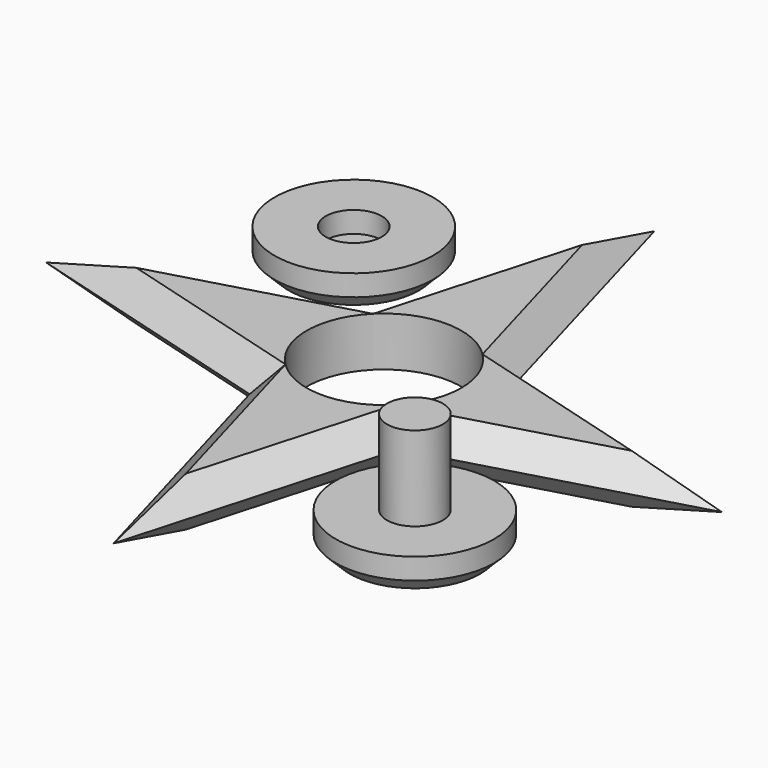
from build123d import *

# Parameters (mm, degrees)
F0_R          = 11
F1_DEPTH      = 7
F2_T4_DEPTH   = 56.8703573637
F2_T9_DEPTH   = 56.8703573637
F2_T14_DEPTH  = 56.8703573637
F2_T19_DEPTH  = 56.8703573637
F2_T24_DEPTH  = 56.8703573637
F2_T29_DEPTH  = 56.8703573637
F2_T34_DEPTH  = 56.8703573637
F2_T39_DEPTH  = 56.8703573637
F2_T44_DEPTH  = 56.8703573637
F2_T49_DEPTH  = 56.8703573637
F2_T54_DEPTH  = 56.8703573637
F2_T59_DEPTH  = 56.8703573637
F2_T64_DEPTH  = 56.8703573637
F2_T69_DEPTH  = 56.8703573637
F2_T74_DEPTH  = 56.8703573637
F2_T79_DEPTH  = 56.8703573637
F2_T85_DEPTH  = 56.8703573637
F2_T89_DEPTH  = 56.8703573637
F2_T96_DEPTH  = 56.8703573637
F2_T100_DEPTH = 56.8703573637
F2_T107_DEPTH = 56.8703573637
F2_T111_DEPTH = 56.8703573637
F2_T118_DEPTH = 56.8703573637
F2_T122_DEPTH = 56.8703573637
F2_T129_DEPTH = 56.8703573637
F2_T133_DEPTH = 56.8703573637
F2_T140_DEPTH = 56.8703573637
F2_T144_DEPTH = 56.8703573637
F2_T151_DEPTH = 56.8703573637
F2_T155_DEPTH = 56.8703573637
F2_T162_DEPTH = 56.8703573637
F2_T166_DEPTH = 56.8703573637
F3_R          = 11.25
F4_DEPTH      = 5
F5_R          = 3.98
F6_DEPTH      = 12
F7_SIZE       = 2
F8_R          = 11.25
F9_DEPTH      = 5
F10_R         = 3.98
F11_DEPTH     = 3
F12_SIZE      = 2


# Not quite as in the source:
# - a fillet or chamfer that OpenCascade refuses, or shapes differently, is made with other operations: its cross-section is extruded or revolved along the edge and cut away or added


with BuildPart() as f1:
    # F0 (on Top) → F1 (new body)
    with BuildSketch(Plane.XY):
        Polygon((-10.6066017178, 10.6066017178), (-48, 0), (-10.6066017178, -10.6066017178), (0, -48), (10.6066017178, -10.6066017178), (48, 0), (10.6066017178, 10.6066017178), (0, 48), align=None)
        Circle(F0_R, mode=Mode.SUBTRACT)
    extrude(amount=F1_DEPTH)

    # F2: chamfer of 3.5 on 16 edges, made by hand


with BuildPart() as f2_tool2:
    # F2_s3 → F2_t4 (new body)
    with BuildSketch(Plane(origin=(15.0574910401, 53.0849347014, 0), x_dir=(0, 0, 1), z_dir=(-0.2728837196, -0.9620470236, 0))):
        Polygon((3.5, 13.0984185422), (7, 9.5984185422), (7, 13.0984185422), align=None)
    extrude(amount=F2_T4_DEPTH)

    split(bisect_by=Plane(origin=(-3.574345173, 12.601294572, 0), x_dir=(0, 0, 1), z_dir=(-0.2728837196, 0.9620470236, 0)), keep=Keep.TOP)


with BuildPart() as f1_1:
    add(f1.part)

    # F2_t1: cut F2_tool2
    add(f2_tool2.part, mode=Mode.SUBTRACT)


with BuildPart() as f2_tool7:
    # F2_s8 → F2_t9 (new body)
    with BuildSketch(Plane(origin=(0.4615036139, -1.6270233297, 0), x_dir=(0, 0, 1), z_dir=(-0.2728837196, 0.9620470236, 0))):
        Polygon((3.5, 13.0984185422), (7, 9.5984185422), (7, 13.0984185422), align=None)
    extrude(amount=F2_T9_DEPTH)

    split(bisect_by=Plane(origin=(3.574345173, 12.601294572, 0), x_dir=(0, 0, 1), z_dir=(0.2728837196, 0.9620470236, 0)), keep=Keep.TOP)


with BuildPart() as f1_2:
    add(f1_1.part)

    # F2_t6: cut F2_tool7
    add(f2_tool7.part, mode=Mode.SUBTRACT)


with BuildPart() as f2_tool12:
    # F2_s13 → F2_t14 (new body)
    with BuildSketch(Plane(origin=(53.0849347014, -15.0574910401, 0), x_dir=(0, 0, 1), z_dir=(-0.9620470236, 0.2728837196, 0))):
        Polygon((3.5, 13.0984185422), (7, 9.5984185422), (7, 13.0984185422), align=None)
    extrude(amount=F2_T14_DEPTH)

    split(bisect_by=Plane(origin=(12.601294572, 3.574345173, 0), x_dir=(0, 0, 1), z_dir=(0.9620470236, 0.2728837196, 0)), keep=Keep.TOP)


with BuildPart() as f1_3:
    add(f1_2.part)

    # F2_t11: cut F2_tool12
    add(f2_tool12.part, mode=Mode.SUBTRACT)


with BuildPart() as f2_tool17:
    # F2_s18 → F2_t19 (new body)
    with BuildSketch(Plane(origin=(-1.6270233297, -0.4615036139, 0), x_dir=(0, 0, 1), z_dir=(0.9620470236, 0.2728837196, 0))):
        Polygon((3.5, 13.0984185422), (7, 9.5984185422), (7, 13.0984185422), align=None)
    extrude(amount=F2_T19_DEPTH)

    split(bisect_by=Plane(origin=(12.601294572, -3.574345173, 0), x_dir=(0, 0, 1), z_dir=(0.9620470236, -0.2728837196, 0)), keep=Keep.TOP)


with BuildPart() as f1_4:
    add(f1_3.part)

    # F2_t16: cut F2_tool17
    add(f2_tool17.part, mode=Mode.SUBTRACT)


with BuildPart() as f2_tool22:
    # F2_s23 → F2_t24 (new body)
    with BuildSketch(Plane(origin=(-15.0574910401, -53.0849347014, 0), x_dir=(0, 0, 1), z_dir=(0.2728837196, 0.9620470236, 0))):
        Polygon((3.5, 13.0984185422), (7, 9.5984185422), (7, 13.0984185422), align=None)
    extrude(amount=F2_T24_DEPTH)

    split(bisect_by=Plane(origin=(3.574345173, -12.601294572, 0), x_dir=(0, 0, 1), z_dir=(0.2728837196, -0.9620470236, 0)), keep=Keep.TOP)


with BuildPart() as f1_5:
    add(f1_4.part)

    # F2_t21: cut F2_tool22
    add(f2_tool22.part, mode=Mode.SUBTRACT)


with BuildPart() as f2_tool27:
    # F2_s28 → F2_t29 (new body)
    with BuildSketch(Plane(origin=(-0.4615036139, 1.6270233297, 0), x_dir=(0, 0, 1), z_dir=(0.2728837196, -0.9620470236, 0))):
        Polygon((3.5, 13.0984185422), (7, 9.5984185422), (7, 13.0984185422), align=None)
    extrude(amount=F2_T29_DEPTH)

    split(bisect_by=Plane(origin=(-3.574345173, -12.601294572, 0), x_dir=(0, 0, 1), z_dir=(-0.2728837196, -0.9620470236, 0)), keep=Keep.TOP)


with BuildPart() as f1_6:
    add(f1_5.part)

    # F2_t26: cut F2_tool27
    add(f2_tool27.part, mode=Mode.SUBTRACT)


with BuildPart() as f2_tool32:
    # F2_s33 → F2_t34 (new body)
    with BuildSketch(Plane(origin=(-53.0849347014, 15.0574910401, 0), x_dir=(0, 0, 1), z_dir=(0.9620470236, -0.2728837196, 0))):
        Polygon((3.5, 13.0984185422), (7, 9.5984185422), (7, 13.0984185422), align=None)
    extrude(amount=F2_T34_DEPTH)

    split(bisect_by=Plane(origin=(-12.601294572, -3.574345173, 0), x_dir=(0, 0, 1), z_dir=(-0.9620470236, -0.2728837196, 0)), keep=Keep.TOP)


with BuildPart() as f1_7:
    add(f1_6.part)

    # F2_t31: cut F2_tool32
    add(f2_tool32.part, mode=Mode.SUBTRACT)


with BuildPart() as f2_tool37:
    # F2_s38 → F2_t39 (new body)
    with BuildSketch(Plane(origin=(1.6270233297, 0.4615036139, 0), x_dir=(0, 0, 1), z_dir=(-0.9620470236, -0.2728837196, 0))):
        Polygon((3.5, 13.0984185422), (7, 9.5984185422), (7, 13.0984185422), align=None)
    extrude(amount=F2_T39_DEPTH)

    split(bisect_by=Plane(origin=(-12.601294572, 3.574345173, 0), x_dir=(0, 0, 1), z_dir=(-0.9620470236, 0.2728837196, 0)), keep=Keep.TOP)


with BuildPart() as f1_8:
    add(f1_7.part)

    # F2_t36: cut F2_tool37
    add(f2_tool37.part, mode=Mode.SUBTRACT)


with BuildPart() as f2_tool42:
    # F2_s43 → F2_t44 (new body)
    with BuildSketch(Plane(origin=(-53.0849347014, 15.0574910401, 0), x_dir=(0, 0, 1), z_dir=(0.9620470236, -0.2728837196, 0))):
        Polygon((3.5, 13.0984185422), (0, 9.5984185422), (0, 13.0984185422), align=None)
    extrude(amount=F2_T44_DEPTH)

    split(bisect_by=Plane(origin=(-12.601294572, -3.574345173, 0), x_dir=(0, 0, 1), z_dir=(-0.9620470236, -0.2728837196, 0)), keep=Keep.TOP)


with BuildPart() as f1_9:
    add(f1_8.part)

    # F2_t41: cut F2_tool42
    add(f2_tool42.part, mode=Mode.SUBTRACT)


with BuildPart() as f2_tool47:
    # F2_s48 → F2_t49 (new body)
    with BuildSketch(Plane(origin=(1.6270233297, 0.4615036139, 0), x_dir=(0, 0, 1), z_dir=(-0.9620470236, -0.2728837196, 0))):
        Polygon((3.5, 13.0984185422), (0, 9.5984185422), (0, 13.0984185422), align=None)
    extrude(amount=F2_T49_DEPTH)

    split(bisect_by=Plane(origin=(-12.601294572, 3.574345173, 0), x_dir=(0, 0, 1), z_dir=(-0.9620470236, 0.2728837196, 0)), keep=Keep.TOP)


with BuildPart() as f1_10:
    add(f1_9.part)

    # F2_t46: cut F2_tool47
    add(f2_tool47.part, mode=Mode.SUBTRACT)


with BuildPart() as f2_tool52:
    # F2_s53 → F2_t54 (new body)
    with BuildSketch(Plane(origin=(15.0574910401, 53.0849347014, 0), x_dir=(0, 0, 1), z_dir=(-0.2728837196, -0.9620470236, 0))):
        Polygon((3.5, 13.0984185422), (0, 9.5984185422), (0, 13.0984185422), align=None)
    extrude(amount=F2_T54_DEPTH)

    split(bisect_by=Plane(origin=(-3.574345173, 12.601294572, 0), x_dir=(0, 0, 1), z_dir=(-0.2728837196, 0.9620470236, 0)), keep=Keep.TOP)


with BuildPart() as f1_11:
    add(f1_10.part)

    # F2_t51: cut F2_tool52
    add(f2_tool52.part, mode=Mode.SUBTRACT)


with BuildPart() as f2_tool57:
    # F2_s58 → F2_t59 (new body)
    with BuildSketch(Plane(origin=(-0.4615036139, 1.6270233297, 0), x_dir=(0, 0, 1), z_dir=(0.2728837196, -0.9620470236, 0))):
        Polygon((3.5, 13.0984185422), (0, 9.5984185422), (0, 13.0984185422), align=None)
    extrude(amount=F2_T59_DEPTH)

    split(bisect_by=Plane(origin=(-3.574345173, -12.601294572, 0), x_dir=(0, 0, 1), z_dir=(-0.2728837196, -0.9620470236, 0)), keep=Keep.TOP)


with BuildPart() as f1_12:
    add(f1_11.part)

    # F2_t56: cut F2_tool57
    add(f2_tool57.part, mode=Mode.SUBTRACT)


with BuildPart() as f2_tool62:
    # F2_s63 → F2_t64 (new body)
    with BuildSketch(Plane(origin=(-15.0574910401, -53.0849347014, 0), x_dir=(0, 0, 1), z_dir=(0.2728837196, 0.9620470236, 0))):
        Polygon((3.5, 13.0984185422), (0, 9.5984185422), (0, 13.0984185422), align=None)
    extrude(amount=F2_T64_DEPTH)

    split(bisect_by=Plane(origin=(3.574345173, -12.601294572, 0), x_dir=(0, 0, 1), z_dir=(0.2728837196, -0.9620470236, 0)), keep=Keep.TOP)


with BuildPart() as f1_13:
    add(f1_12.part)

    # F2_t61: cut F2_tool62
    add(f2_tool62.part, mode=Mode.SUBTRACT)


with BuildPart() as f2_tool67:
    # F2_s68 → F2_t69 (new body)
    with BuildSketch(Plane(origin=(-1.6270233297, -0.4615036139, 0), x_dir=(0, 0, 1), z_dir=(0.9620470236, 0.2728837196, 0))):
        Polygon((3.5, 13.0984185422), (0, 9.5984185422), (0, 13.0984185422), align=None)
    extrude(amount=F2_T69_DEPTH)

    split(bisect_by=Plane(origin=(12.601294572, -3.574345173, 0), x_dir=(0, 0, 1), z_dir=(0.9620470236, -0.2728837196, 0)), keep=Keep.TOP)


with BuildPart() as f1_14:
    add(f1_13.part)

    # F2_t66: cut F2_tool67
    add(f2_tool67.part, mode=Mode.SUBTRACT)


with BuildPart() as f2_tool72:
    # F2_s73 → F2_t74 (new body)
    with BuildSketch(Plane(origin=(53.0849347014, -15.0574910401, 0), x_dir=(0, 0, 1), z_dir=(-0.9620470236, 0.2728837196, 0))):
        Polygon((3.5, 13.0984185422), (0, 9.5984185422), (0, 13.0984185422), align=None)
    extrude(amount=F2_T74_DEPTH)

    split(bisect_by=Plane(origin=(12.601294572, 3.574345173, 0), x_dir=(0, 0, 1), z_dir=(0.9620470236, 0.2728837196, 0)), keep=Keep.TOP)


with BuildPart() as f1_15:
    add(f1_14.part)

    # F2_t71: cut F2_tool72
    add(f2_tool72.part, mode=Mode.SUBTRACT)


with BuildPart() as f2_tool77:
    # F2_s78 → F2_t79 (new body)
    with BuildSketch(Plane(origin=(0.4615036139, -1.6270233297, 0), x_dir=(0, 0, 1), z_dir=(-0.2728837196, 0.9620470236, 0))):
        Polygon((3.5, 13.0984185422), (0, 9.5984185422), (0, 13.0984185422), align=None)
    extrude(amount=F2_T79_DEPTH)

    split(bisect_by=Plane(origin=(3.574345173, 12.601294572, 0), x_dir=(0, 0, 1), z_dir=(0.2728837196, 0.9620470236, 0)), keep=Keep.TOP)


with BuildPart() as f1_16:
    add(f1_15.part)

    # F2_t76: cut F2_tool77
    add(f2_tool77.part, mode=Mode.SUBTRACT)


with BuildPart() as f2_tool83:
    # F2_s84 → F2_t85 (new body)
    with BuildSketch(Plane(origin=(1.6270233297, 0.4615036139, 0), x_dir=(0, 0, 1), z_dir=(-0.9620470236, -0.2728837196, 0))):
        Polygon((3.5, 13.0984185422), (7, 9.5984185422), (7, 13.0984185422), align=None)
    extrude(amount=F2_T85_DEPTH)

    split(bisect_by=Plane(origin=(-12.601294572, 3.574345173, 0), x_dir=(0, 0, 1), z_dir=(0.9620470236, -0.2728837196, 0)), keep=Keep.TOP)


with BuildPart() as f2_tool87:
    # F2_s88 → F2_t89 (new body)
    with BuildSketch(Plane(origin=(15.0574910401, 53.0849347014, 0), x_dir=(0, 0, 1), z_dir=(-0.2728837196, -0.9620470236, 0))):
        Polygon((3.5, 13.0984185422), (7, 9.5984185422), (7, 13.0984185422), align=None)
    extrude(amount=F2_T89_DEPTH)

    split(bisect_by=Plane(origin=(-3.574345173, 12.601294572, 0), x_dir=(0, 0, 1), z_dir=(0.2728837196, -0.9620470236, 0)), keep=Keep.TOP)


with BuildPart() as f2_tool83_1:
    add(f2_tool83.part)

    # F2_t91: intersect F2_tool87
    add(f2_tool87.part, mode=Mode.INTERSECT)


with BuildPart() as f1_17:
    add(f1_16.part)

    # F2_t81: cut F2_tool83
    add(f2_tool83_1.part, mode=Mode.SUBTRACT)


with BuildPart() as f2_tool94:
    # F2_s95 → F2_t96 (new body)
    with BuildSketch(Plane(origin=(53.0849347014, -15.0574910401, 0), x_dir=(0, 0, 1), z_dir=(-0.9620470236, 0.2728837196, 0))):
        Polygon((3.5, 13.0984185422), (7, 9.5984185422), (7, 13.0984185422), align=None)
    extrude(amount=F2_T96_DEPTH)

    split(bisect_by=Plane(origin=(12.601294572, 3.574345173, 0), x_dir=(0, 0, 1), z_dir=(-0.9620470236, -0.2728837196, 0)), keep=Keep.TOP)


with BuildPart() as f2_tool98:
    # F2_s99 → F2_t100 (new body)
    with BuildSketch(Plane(origin=(0.4615036139, -1.6270233297, 0), x_dir=(0, 0, 1), z_dir=(-0.2728837196, 0.9620470236, 0))):
        Polygon((3.5, 13.0984185422), (7, 9.5984185422), (7, 13.0984185422), align=None)
    extrude(amount=F2_T100_DEPTH)

    split(bisect_by=Plane(origin=(3.574345173, 12.601294572, 0), x_dir=(0, 0, 1), z_dir=(-0.2728837196, -0.9620470236, 0)), keep=Keep.TOP)


with BuildPart() as f2_tool94_1:
    add(f2_tool94.part)

    # F2_t102: intersect F2_tool98
    add(f2_tool98.part, mode=Mode.INTERSECT)


with BuildPart() as f1_18:
    add(f1_17.part)

    # F2_t92: cut F2_tool94
    add(f2_tool94_1.part, mode=Mode.SUBTRACT)


with BuildPart() as f2_tool105:
    # F2_s106 → F2_t107 (new body)
    with BuildSketch(Plane(origin=(-15.0574910401, -53.0849347014, 0), x_dir=(0, 0, 1), z_dir=(0.2728837196, 0.9620470236, 0))):
        Polygon((3.5, 13.0984185422), (7, 9.5984185422), (7, 13.0984185422), align=None)
    extrude(amount=F2_T107_DEPTH)

    split(bisect_by=Plane(origin=(3.574345173, -12.601294572, 0), x_dir=(0, 0, 1), z_dir=(-0.2728837196, 0.9620470236, 0)), keep=Keep.TOP)


with BuildPart() as f2_tool109:
    # F2_s110 → F2_t111 (new body)
    with BuildSketch(Plane(origin=(-1.6270233297, -0.4615036139, 0), x_dir=(0, 0, 1), z_dir=(0.9620470236, 0.2728837196, 0))):
        Polygon((3.5, 13.0984185422), (7, 9.5984185422), (7, 13.0984185422), align=None)
    extrude(amount=F2_T111_DEPTH)

    split(bisect_by=Plane(origin=(12.601294572, -3.574345173, 0), x_dir=(0, 0, 1), z_dir=(-0.9620470236, 0.2728837196, 0)), keep=Keep.TOP)


with BuildPart() as f2_tool105_1:
    add(f2_tool105.part)

    # F2_t113: intersect F2_tool109
    add(f2_tool109.part, mode=Mode.INTERSECT)


with BuildPart() as f1_19:
    add(f1_18.part)

    # F2_t103: cut F2_tool105
    add(f2_tool105_1.part, mode=Mode.SUBTRACT)


with BuildPart() as f2_tool116:
    # F2_s117 → F2_t118 (new body)
    with BuildSketch(Plane(origin=(-53.0849347014, 15.0574910401, 0), x_dir=(0, 0, 1), z_dir=(0.9620470236, -0.2728837196, 0))):
        Polygon((3.5, 13.0984185422), (7, 9.5984185422), (7, 13.0984185422), align=None)
    extrude(amount=F2_T118_DEPTH)

    split(bisect_by=Plane(origin=(-12.601294572, -3.574345173, 0), x_dir=(0, 0, 1), z_dir=(0.9620470236, 0.2728837196, 0)), keep=Keep.TOP)


with BuildPart() as f2_tool120:
    # F2_s121 → F2_t122 (new body)
    with BuildSketch(Plane(origin=(-0.4615036139, 1.6270233297, 0), x_dir=(0, 0, 1), z_dir=(0.2728837196, -0.9620470236, 0))):
        Polygon((3.5, 13.0984185422), (7, 9.5984185422), (7, 13.0984185422), align=None)
    extrude(amount=F2_T122_DEPTH)

    split(bisect_by=Plane(origin=(-3.574345173, -12.601294572, 0), x_dir=(0, 0, 1), z_dir=(0.2728837196, 0.9620470236, 0)), keep=Keep.TOP)


with BuildPart() as f2_tool116_1:
    add(f2_tool116.part)

    # F2_t124: intersect F2_tool120
    add(f2_tool120.part, mode=Mode.INTERSECT)


with BuildPart() as f1_20:
    add(f1_19.part)

    # F2_t114: cut F2_tool116
    add(f2_tool116_1.part, mode=Mode.SUBTRACT)


with BuildPart() as f2_tool127:
    # F2_s128 → F2_t129 (new body)
    with BuildSketch(Plane(origin=(-53.0849347014, 15.0574910401, 0), x_dir=(0, 0, 1), z_dir=(0.9620470236, -0.2728837196, 0))):
        Polygon((3.5, 13.0984185422), (0, 9.5984185422), (0, 13.0984185422), align=None)
    extrude(amount=F2_T129_DEPTH)

    split(bisect_by=Plane(origin=(-12.601294572, -3.574345173, 0), x_dir=(0, 0, 1), z_dir=(0.9620470236, 0.2728837196, 0)), keep=Keep.TOP)


with BuildPart() as f2_tool131:
    # F2_s132 → F2_t133 (new body)
    with BuildSketch(Plane(origin=(-0.4615036139, 1.6270233297, 0), x_dir=(0, 0, 1), z_dir=(0.2728837196, -0.9620470236, 0))):
        Polygon((3.5, 13.0984185422), (0, 9.5984185422), (0, 13.0984185422), align=None)
    extrude(amount=F2_T133_DEPTH)

    split(bisect_by=Plane(origin=(-3.574345173, -12.601294572, 0), x_dir=(0, 0, 1), z_dir=(0.2728837196, 0.9620470236, 0)), keep=Keep.TOP)


with BuildPart() as f2_tool127_1:
    add(f2_tool127.part)

    # F2_t135: intersect F2_tool131
    add(f2_tool131.part, mode=Mode.INTERSECT)


with BuildPart() as f1_21:
    add(f1_20.part)

    # F2_t125: cut F2_tool127
    add(f2_tool127_1.part, mode=Mode.SUBTRACT)


with BuildPart() as f2_tool138:
    # F2_s139 → F2_t140 (new body)
    with BuildSketch(Plane(origin=(1.6270233297, 0.4615036139, 0), x_dir=(0, 0, 1), z_dir=(-0.9620470236, -0.2728837196, 0))):
        Polygon((3.5, 13.0984185422), (0, 9.5984185422), (0, 13.0984185422), align=None)
    extrude(amount=F2_T140_DEPTH)

    split(bisect_by=Plane(origin=(-12.601294572, 3.574345173, 0), x_dir=(0, 0, 1), z_dir=(0.9620470236, -0.2728837196, 0)), keep=Keep.TOP)


with BuildPart() as f2_tool142:
    # F2_s143 → F2_t144 (new body)
    with BuildSketch(Plane(origin=(15.0574910401, 53.0849347014, 0), x_dir=(0, 0, 1), z_dir=(-0.2728837196, -0.9620470236, 0))):
        Polygon((3.5, 13.0984185422), (0, 9.5984185422), (0, 13.0984185422), align=None)
    extrude(amount=F2_T144_DEPTH)

    split(bisect_by=Plane(origin=(-3.574345173, 12.601294572, 0), x_dir=(0, 0, 1), z_dir=(0.2728837196, -0.9620470236, 0)), keep=Keep.TOP)


with BuildPart() as f2_tool138_1:
    add(f2_tool138.part)

    # F2_t146: intersect F2_tool142
    add(f2_tool142.part, mode=Mode.INTERSECT)


with BuildPart() as f1_22:
    add(f1_21.part)

    # F2_t136: cut F2_tool138
    add(f2_tool138_1.part, mode=Mode.SUBTRACT)


with BuildPart() as f2_tool149:
    # F2_s150 → F2_t151 (new body)
    with BuildSketch(Plane(origin=(-15.0574910401, -53.0849347014, 0), x_dir=(0, 0, 1), z_dir=(0.2728837196, 0.9620470236, 0))):
        Polygon((3.5, 13.0984185422), (0, 9.5984185422), (0, 13.0984185422), align=None)
    extrude(amount=F2_T151_DEPTH)

    split(bisect_by=Plane(origin=(3.574345173, -12.601294572, 0), x_dir=(0, 0, 1), z_dir=(-0.2728837196, 0.9620470236, 0)), keep=Keep.TOP)


with BuildPart() as f2_tool153:
    # F2_s154 → F2_t155 (new body)
    with BuildSketch(Plane(origin=(-1.6270233297, -0.4615036139, 0), x_dir=(0, 0, 1), z_dir=(0.9620470236, 0.2728837196, 0))):
        Polygon((3.5, 13.0984185422), (0, 9.5984185422), (0, 13.0984185422), align=None)
    extrude(amount=F2_T155_DEPTH)

    split(bisect_by=Plane(origin=(12.601294572, -3.574345173, 0), x_dir=(0, 0, 1), z_dir=(-0.9620470236, 0.2728837196, 0)), keep=Keep.TOP)


with BuildPart() as f2_tool149_1:
    add(f2_tool149.part)

    # F2_t157: intersect F2_tool153
    add(f2_tool153.part, mode=Mode.INTERSECT)


with BuildPart() as f1_23:
    add(f1_22.part)

    # F2_t147: cut F2_tool149
    add(f2_tool149_1.part, mode=Mode.SUBTRACT)


with BuildPart() as f2_tool160:
    # F2_s161 → F2_t162 (new body)
    with BuildSketch(Plane(origin=(53.0849347014, -15.0574910401, 0), x_dir=(0, 0, 1), z_dir=(-0.9620470236, 0.2728837196, 0))):
        Polygon((3.5, 13.0984185422), (0, 9.5984185422), (0, 13.0984185422), align=None)
    extrude(amount=F2_T162_DEPTH)

    split(bisect_by=Plane(origin=(12.601294572, 3.574345173, 0), x_dir=(0, 0, 1), z_dir=(-0.9620470236, -0.2728837196, 0)), keep=Keep.TOP)


with BuildPart() as f2_tool164:
    # F2_s165 → F2_t166 (new body)
    with BuildSketch(Plane(origin=(0.4615036139, -1.6270233297, 0), x_dir=(0, 0, 1), z_dir=(-0.2728837196, 0.9620470236, 0))):
        Polygon((3.5, 13.0984185422), (0, 9.5984185422), (0, 13.0984185422), align=None)
    extrude(amount=F2_T166_DEPTH)

    split(bisect_by=Plane(origin=(3.574345173, 12.601294572, 0), x_dir=(0, 0, 1), z_dir=(-0.2728837196, -0.9620470236, 0)), keep=Keep.TOP)


with BuildPart() as f2_tool160_1:
    add(f2_tool160.part)

    # F2_t168: intersect F2_tool164
    add(f2_tool164.part, mode=Mode.INTERSECT)


with BuildPart() as f1_24:
    add(f1_23.part)

    # F2_t158: cut F2_tool160
    add(f2_tool160_1.part, mode=Mode.SUBTRACT)


with BuildPart() as f4:
    # F3 (on Top) → F4 (new body)
    with BuildSketch(Plane.XY):
        with Locations((-50.1265861094, 32.8955687582)):
            Circle(F3_R)
    extrude(amount=F4_DEPTH)

    # F5 (on face) → F6 (join)
    with BuildSketch(Plane.XY.offset(5)):
        with Locations((-50.1265861094, 32.8955687582)):
            Circle(F5_R)
    extrude(amount=F6_DEPTH)

    # F7
    f7_edges = [f4.edges().sort_by_distance(p)[0] for p in [
        (-61.376586, 32.895569, 0),
    ]]
    chamfer(f7_edges, length=F7_SIZE)


with BuildPart() as f9:
    # F8 (on Top) → F9 (new body)
    with BuildSketch(Plane.XY):
        with Locations((-24.9479543418, 34.8169021308)):
            Circle(F8_R)
    extrude(amount=F9_DEPTH)

    # F10 (on face) → F11 (cut)
    with BuildSketch(Plane.XY.offset(5)):
        with Locations((-24.9479543418, 34.8169021308)):
            Circle(F10_R)
    extrude(amount=-F11_DEPTH, mode=Mode.SUBTRACT)

    # F12
    f12_edges = [f9.edges().sort_by_distance(p)[0] for p in [
        (-36.197954, 34.816902, 0),
    ]]
    chamfer(f12_edges, length=F12_SIZE)


with BuildPart() as f4_1:
    # F13: moved
    add(f4.part.moved(Location((73, -56, 0))))


with BuildPart() as f9_1:
    # F14: moved
    add(f9.part.moved(Location((0, -9, 0))))


solid = Compound([f1_24.part, f4_1.part, f9_1.part])
